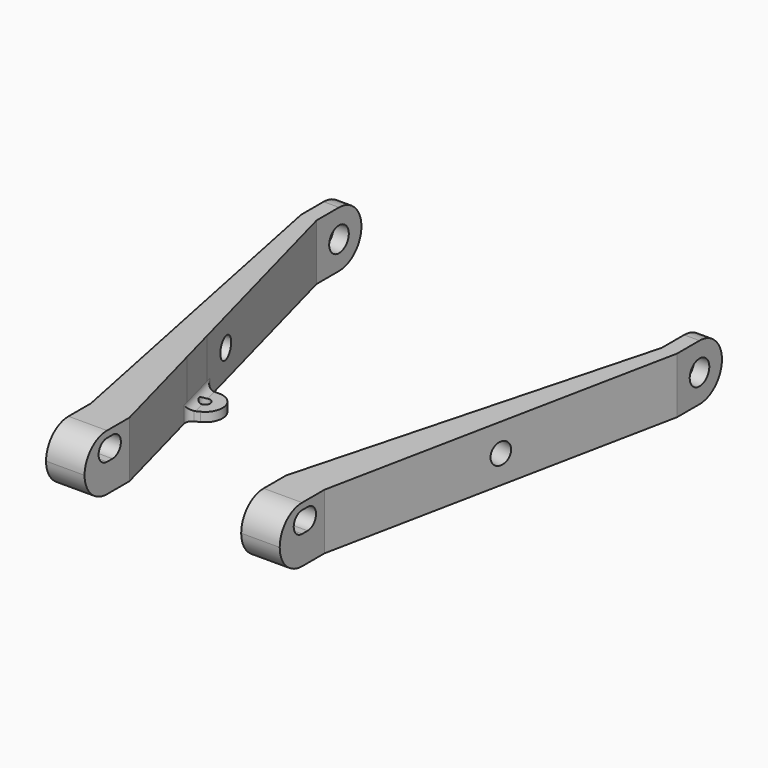
from build123d import *

# Parameters (mm, degrees)
F1_DEPTH        = 8
F0_W            = 2.2
F0_H            = 8
F0_W_2          = 5.5
F0_R            = 0.75
F2_DEPTH        = 1.3
F3_R            = 1.75
F4_DEPTH        = 53.6778461441
F5_R            = 1.5
F6_DEPTH        = 25
F7_R            = 1.5
F8_DEPTH        = 25
F9_R            = 3.99999
F9_2_R          = 3.99999
F10_T1_DEPTH    = 1.3
F10_T6_DEPTH    = 10.6165464639
F10_S9_R        = 0.75
F10_T10_DEPTH   = 7
F10_T15_DEPTH   = 10.6165464639
F10_T19_DEPTH   = 3.3290625116
F10_T26_DEPTH   = 3.2183174699
F10_T30_DEPTH   = 10.6165464639
F10_2_T1_DEPTH  = 1.3
F10_2_T6_DEPTH  = 10.6165464639
F10_2_S9_R      = 0.75
F10_2_T10_DEPTH = 7
F10_2_T15_DEPTH = 3.3290625116
F10_2_T19_DEPTH = 10.6165464639
F10_2_T26_DEPTH = 10.6165464639
F10_2_T30_DEPTH = 3.2183174699


# Not quite as in the source:
# - a fillet or chamfer that OpenCascade refuses, or shapes differently, is made with other operations: its cross-section is extruded or revolved along the edge and cut away or added
# - a fillet or chamfer is up to 0.001 mm smaller than in the source, because OpenCascade refuses the exact size


with BuildPart() as f1:
    # F0 (on Top) → F1 (new body)
    with BuildSketch(Plane.XY):
        Polygon((38.5682557988, 62.228142967), (38.5682557988, 54.228142967), (30.6936795925, 24.8398244771), (29.2400103999, 19.414657193), (25.1096654534, 4), (25.1096654534, -4), (30.6096654534, -4), (30.6096654534, 4), (40.7682557988, 54.228142967), (40.7682557988, 62.228142967), align=None)
    extrude(amount=F1_DEPTH)

    # F0 (on Top) → F2, piece 2 (join)
    with BuildSketch(Plane.XY):
        with BuildLine():
            Line((29.2400103999, 19.414657193), (30.6936795925, 24.8398244771))
            Line((30.6936795925, 24.8398244771), (29.1367222868, 24.8398244771))
            ThreePointArc((29.1367222868, 24.8398244771), (26.5762608106, 22.9963479894), (27.8596654534, 20.1141195019))
            Line((27.8596654534, 20.1141195019), (29.2400103999, 19.414657193))
        make_face()
        with Locations((28.9896899666, 22.3441519231)):
            Circle(F0_R, mode=Mode.SUBTRACT)
    extrude(amount=F2_DEPTH)


with BuildPart() as f1b:
    # F0 (on Top) → F1, piece 2 (new body)
    with BuildSketch(Plane.XY):
        Polygon((-2.75, 4), (2.75, 4), (-1.3803449465, 19.414657193), (-2.834014139, 24.8398244771), (-10.7085903453, 54.228142967), (-12.9085903453, 54.228142967), align=None)
        with Locations((-11.8085903453, 58.228142967)):
            Rectangle(F0_W, F0_H)
        Rectangle(F0_W_2, F0_H)
    extrude(amount=F1_DEPTH)

    # F0 (on Top) → F2 (join)
    with BuildSketch(Plane.XY):
        with BuildLine():
            Line((-2.834014139, 24.8398244771), (-1.3803449465, 19.414657193))
            Line((-1.3803449465, 19.414657193), (0, 20.1141195019))
            ThreePointArc((0, 20.1141195019), (1.2834046428, 22.9963479894), (-1.2770568333, 24.8398244771))
            Line((-1.2770568333, 24.8398244771), (-2.834014139, 24.8398244771))
        make_face()
        with Locations((-1.1300245132, 22.3441519231)):
            Circle(F0_R, mode=Mode.SUBTRACT)
    extrude(amount=F2_DEPTH)


with BuildPart() as f4_tool:
    # F3 (on face) → F4 (new body, through all)
    with BuildSketch(Plane(origin=(-12.9085903453, 0, 0), x_dir=(0, -1, 0), z_dir=(-1, 0, 0))):
        with BuildLine():
            Line((-0.9781668196, 4.0648819543), (0, 4.0648819543))
            ThreePointArc((0, 4.0648819543), (1.5, 5.5648819543), (0, 7.0648819543))
            Line((0, 7.0648819543), (-0.9781668196, 7.0648819543))
            ThreePointArc((-0.9781668196, 7.0648819543), (-2.4781668196, 5.5648819543), (-0.9781668196, 4.0648819543))
        make_face()
        with Locations((-58.228142967, 4)):
            Circle(F3_R)
    extrude(amount=-F4_DEPTH)


with BuildPart() as f1_1:
    add(f1.part)

    # F4: cut by f4_tool
    add(f4_tool.part, mode=Mode.SUBTRACT)

    # F7 (on face) → F8 (cut)
    with BuildSketch(Plane(origin=(28.629586428, -5.7903044608, 0), x_dir=(0.1982352359, 0.9801544732, 0), z_dir=(0.9801544732, -0.1982352359, 0))):
        with Locations((35.611096924, 4)):
            Circle(F7_R)
    extrude(amount=-F8_DEPTH, mode=Mode.SUBTRACT)

    # F9 (radius 4 in the source; OpenCascade refuses exactly that, so slightly less here)
    f9_edges = [f1_1.edges().sort_by_distance(p)[0] for p in [
        (27.859665, -4, 8),
        (39.668256, 62.228143, 8),
        (39.668256, 62.228143, 0),
        (27.859665, -4, 0),
    ]]
    fillet(f9_edges, radius=F9_R)

    # F10: fillet of radius 1 on 3 edges, made by hand

    # F10_s2 → F10_t1 (join)
    with BuildSketch(Plane.XY):
        with BuildLine():
            ThreePointArc((30.8922784308, 25.581005432), (30.5351140335, 25.0464711368), (29.9263526045, 24.8398244771))
            Line((29.9263526045, 24.8398244771), (30.6936795925, 24.8398244771))
            Line((30.6936795925, 24.8398244771), (30.8922784308, 25.581005432))
        make_face()
        with BuildLine():
            ThreePointArc((29.0299463912, 18.6306876398), (28.9771136296, 19.2972579023), (28.5160303702, 19.7815196533))
            Line((28.5160303702, 19.7815196533), (29.2400103999, 19.414657193))
            Line((29.2400103999, 19.414657193), (29.0299463912, 18.6306876398))
        make_face()
    extrude(amount=F10_T1_DEPTH)


with BuildPart() as f1b_1:
    add(f1b.part)

    # F4: cut by f4_tool
    add(f4_tool.part, mode=Mode.SUBTRACT)

    # F5 (on face) → F6 (cut)
    with BuildSketch(Plane(origin=(-1.8647280633, -0.3771393363, 0), x_dir=(0.1982352359, -0.9801544732, 0), z_dir=(-0.9801544732, -0.1982352359, 0))):
        with Locations((-30.0883295718, 4)):
            Circle(F5_R)
    extrude(amount=-F6_DEPTH, mode=Mode.SUBTRACT)

    # F9#2 (radius 4 in the source; OpenCascade refuses exactly that, so slightly less here)
    f9_2_edges = [f1b_1.edges().sort_by_distance(p)[0] for p in [
        (-11.80859, 62.228143, 8),
        (0, -4, 8),
        (-11.80859, 62.228143, 0),
        (0, -4, 0),
    ]]
    fillet(f9_2_edges, radius=F9_2_R)

    # F10#2: fillet of radius 1 on 3 edges, made by hand

    # F10_2_s2 → F10_2_t1 (join)
    with BuildSketch(Plane.XY):
        with BuildLine():
            ThreePointArc((-1.1702809378, 18.6306876398), (-1.1174481761, 19.2972579023), (-0.6563649168, 19.7815196533))
            Line((-0.6563649168, 19.7815196533), (-1.3803449465, 19.414657193))
            Line((-1.3803449465, 19.414657193), (-1.1702809378, 18.6306876398))
        make_face()
        with BuildLine():
            ThreePointArc((-3.0326129774, 25.581005432), (-2.6754485801, 25.0464711368), (-2.0666871511, 24.8398244771))
            Line((-2.0666871511, 24.8398244771), (-2.834014139, 24.8398244771))
            Line((-2.834014139, 24.8398244771), (-3.0326129774, 25.581005432))
        make_face()
    extrude(amount=F10_2_T1_DEPTH)


with BuildPart() as f10_tool4:
    # F10_s5 → F10_t6 (new body)
    with BuildSketch(Plane(origin=(6.1653259788, 23.0093097982, 0), x_dir=(0, 0, 1), z_dir=(0.2588190451, 0.9659258263, 0))):
        with BuildLine():
            ThreePointArc((2.3, 23.2187981705), (1.5928932188, 22.9259049517), (1.3, 22.2187981705))
            Line((1.3, 22.2187981705), (1.3, 23.2187981705))
            Line((1.3, 23.2187981705), (2.3, 23.2187981705))
        make_face()
    extrude(amount=F10_T6_DEPTH)

    split(bisect_by=Plane.XZ.offset(-24.8398244771), keep=Keep.TOP)

    split(bisect_by=Plane(origin=(13.8020730291, 27.2375244736, 0), x_dir=(0, 0, 1), z_dir=(0.4520098053, 0.8920129685, 0)), keep=Keep.TOP)

    # F10_s9 → F10_t10 (cut, symmetric)
    with BuildSketch(Plane.XY.offset(1.8)):
        with Locations((28.9896899666, 22.3441519231)):
            Circle(F10_S9_R)
    extrude(amount=F10_T10_DEPTH, both=True, mode=Mode.SUBTRACT)


with BuildPart() as f1_2:
    add(f1_1.part)

    # F10_t3: union F10_tool4
    add(f10_tool4.part)


with BuildPart() as f10_tool13:
    # F10_s14 → F10_t15 (new body)
    with BuildSketch(Plane(origin=(6.1653259788, 23.0093097982, 0), x_dir=(0, 0, 1), z_dir=(0.2588190451, 0.9659258263, 0))):
        with BuildLine():
            ThreePointArc((2.3, 23.2187981705), (1.5928932188, 22.9259049517), (1.3, 22.2187981705))
            Line((1.3, 22.2187981705), (1.3, 23.2187981705))
            Line((1.3, 23.2187981705), (2.3, 23.2187981705))
        make_face()
    extrude(amount=F10_T15_DEPTH)

    split(bisect_by=Plane(origin=(13.8020730291, 27.2375244736, 0), x_dir=(0, 0, 1), z_dir=(-0.4520098053, -0.8920129685, 0)), keep=Keep.TOP)


with BuildPart() as f10_tool17:
    # F10_s18 → F10_t19 (new body)
    with BuildSketch(Plane.XY):
        with BuildLine():
            ThreePointArc((29.0299463912, 18.6306876398), (28.9771136296, 19.2972579023), (28.5160303702, 19.7815196533))
            Line((28.5160303702, 19.7815196533), (29.2400103999, 19.414657193))
            Line((29.2400103999, 19.414657193), (29.0299463912, 18.6306876398))
        make_face()
    extrude(amount=F10_T19_DEPTH)

    split(bisect_by=Plane.XY.offset(1.3), keep=Keep.TOP)


with BuildPart() as f10_tool13_1:
    add(f10_tool13.part)

    # F10_t21: intersect F10_tool17
    add(f10_tool17.part, mode=Mode.INTERSECT)


with BuildPart() as f1_3:
    add(f1_2.part)

    # F10_t11: union F10_tool13
    add(f10_tool13_1.part)


with BuildPart() as f10_tool24:
    # F10_s25 → F10_t26 (new body)
    with BuildSketch(Plane.XY):
        with BuildLine():
            ThreePointArc((30.8922784308, 25.581005432), (30.5351140335, 25.0464711368), (29.9263526045, 24.8398244771))
            Line((29.9263526045, 24.8398244771), (30.6936795925, 24.8398244771))
            Line((30.6936795925, 24.8398244771), (30.8922784308, 25.581005432))
        make_face()
    extrude(amount=F10_T26_DEPTH)

    split(bisect_by=Plane.XY.offset(1.3), keep=Keep.TOP)


with BuildPart() as f10_tool28:
    # F10_s29 → F10_t30 (new body)
    with BuildSketch(Plane(origin=(6.1653259788, 23.0093097982, 0), x_dir=(0, 0, 1), z_dir=(0.2588190451, 0.9659258263, 0))):
        with BuildLine():
            ThreePointArc((2.3, 23.2187981705), (1.5928932188, 22.9259049517), (1.3, 22.2187981705))
            Line((1.3, 22.2187981705), (1.3, 23.2187981705))
            Line((1.3, 23.2187981705), (2.3, 23.2187981705))
        make_face()
    extrude(amount=F10_T30_DEPTH)

    split(bisect_by=Plane.XZ.offset(-24.8398244771), keep=Keep.BOTTOM)


with BuildPart() as f10_tool24_1:
    add(f10_tool24.part)

    # F10_t32: intersect F10_tool28
    add(f10_tool28.part, mode=Mode.INTERSECT)


with BuildPart() as f1_4:
    add(f1_3.part)

    # F10_t22: union F10_tool24
    add(f10_tool24_1.part)


with BuildPart() as f10_2_tool4:
    # F10_2_s5 → F10_2_t6 (new body)
    with BuildSketch(Plane(origin=(-7.046846682, 26.2991898504, 0), x_dir=(0, 0, 1), z_dir=(0.2588190451, -0.9659258263, 0))):
        with BuildLine():
            ThreePointArc((2.3, -3.6915722027), (1.5928932188, -3.9844654215), (1.3, -4.6915722027))
            Line((1.3, -4.6915722027), (1.3, -3.6915722027))
            Line((1.3, -3.6915722027), (2.3, -3.6915722027))
        make_face()
    extrude(amount=F10_2_T6_DEPTH)

    split(bisect_by=Plane(origin=(-8.1099849882, 16.0045461381, 0), x_dir=(0, 0, 1), z_dir=(-0.4520098053, 0.8920129685, 0)), keep=Keep.TOP)

    split(bisect_by=Plane.XZ.offset(-24.8398244771), keep=Keep.TOP)

    # F10_2_s9 → F10_2_t10 (cut, symmetric)
    with BuildSketch(Plane.XY.offset(1.8)):
        with Locations((-1.1300245132, 22.3441519231)):
            Circle(F10_2_S9_R)
    extrude(amount=F10_2_T10_DEPTH, both=True, mode=Mode.SUBTRACT)


with BuildPart() as f1b_2:
    add(f1b_1.part)

    # F10_2_t3: union F10_2_tool4
    add(f10_2_tool4.part)


with BuildPart() as f10_2_tool13:
    # F10_2_s14 → F10_2_t15 (new body)
    with BuildSketch(Plane.XY):
        with BuildLine():
            ThreePointArc((-1.1702809378, 18.6306876398), (-1.1174481761, 19.2972579023), (-0.6563649168, 19.7815196533))
            Line((-0.6563649168, 19.7815196533), (-1.3803449465, 19.414657193))
            Line((-1.3803449465, 19.414657193), (-1.1702809378, 18.6306876398))
        make_face()
    extrude(amount=F10_2_T15_DEPTH)

    split(bisect_by=Plane.XY.offset(1.3), keep=Keep.TOP)


with BuildPart() as f10_2_tool17:
    # F10_2_s18 → F10_2_t19 (new body)
    with BuildSketch(Plane(origin=(-7.046846682, 26.2991898504, 0), x_dir=(0, 0, 1), z_dir=(0.2588190451, -0.9659258263, 0))):
        with BuildLine():
            ThreePointArc((2.3, -3.6915722027), (1.5928932188, -3.9844654215), (1.3, -4.6915722027))
            Line((1.3, -4.6915722027), (1.3, -3.6915722027))
            Line((1.3, -3.6915722027), (2.3, -3.6915722027))
        make_face()
    extrude(amount=F10_2_T19_DEPTH)

    split(bisect_by=Plane(origin=(-8.1099849882, 16.0045461381, 0), x_dir=(0, 0, 1), z_dir=(0.4520098053, -0.8920129685, 0)), keep=Keep.TOP)


with BuildPart() as f10_2_tool13_1:
    add(f10_2_tool13.part)

    # F10_2_t21: intersect F10_2_tool17
    add(f10_2_tool17.part, mode=Mode.INTERSECT)


with BuildPart() as f1b_3:
    add(f1b_2.part)

    # F10_2_t11: union F10_2_tool13
    add(f10_2_tool13_1.part)


with BuildPart() as f10_2_tool24:
    # F10_2_s25 → F10_2_t26 (new body)
    with BuildSketch(Plane(origin=(-7.046846682, 26.2991898504, 0), x_dir=(0, 0, 1), z_dir=(0.2588190451, -0.9659258263, 0))):
        with BuildLine():
            ThreePointArc((2.3, -3.6915722027), (1.5928932188, -3.9844654215), (1.3, -4.6915722027))
            Line((1.3, -4.6915722027), (1.3, -3.6915722027))
            Line((1.3, -3.6915722027), (2.3, -3.6915722027))
        make_face()
    extrude(amount=F10_2_T26_DEPTH)

    split(bisect_by=Plane.XZ.offset(-24.8398244771), keep=Keep.BOTTOM)


with BuildPart() as f10_2_tool28:
    # F10_2_s29 → F10_2_t30 (new body)
    with BuildSketch(Plane.XY):
        with BuildLine():
            ThreePointArc((-3.0326129774, 25.581005432), (-2.6754485801, 25.0464711368), (-2.0666871511, 24.8398244771))
            Line((-2.0666871511, 24.8398244771), (-2.834014139, 24.8398244771))
            Line((-2.834014139, 24.8398244771), (-3.0326129774, 25.581005432))
        make_face()
    extrude(amount=F10_2_T30_DEPTH)

    split(bisect_by=Plane.XY.offset(1.3), keep=Keep.TOP)


with BuildPart() as f10_2_tool24_1:
    add(f10_2_tool24.part)

    # F10_2_t32: intersect F10_2_tool28
    add(f10_2_tool28.part, mode=Mode.INTERSECT)


with BuildPart() as f1b_4:
    add(f1b_3.part)

    # F10_2_t22: union F10_2_tool24
    add(f10_2_tool24_1.part)


solid = Compound([f1_4.part, f1b_4.part])
